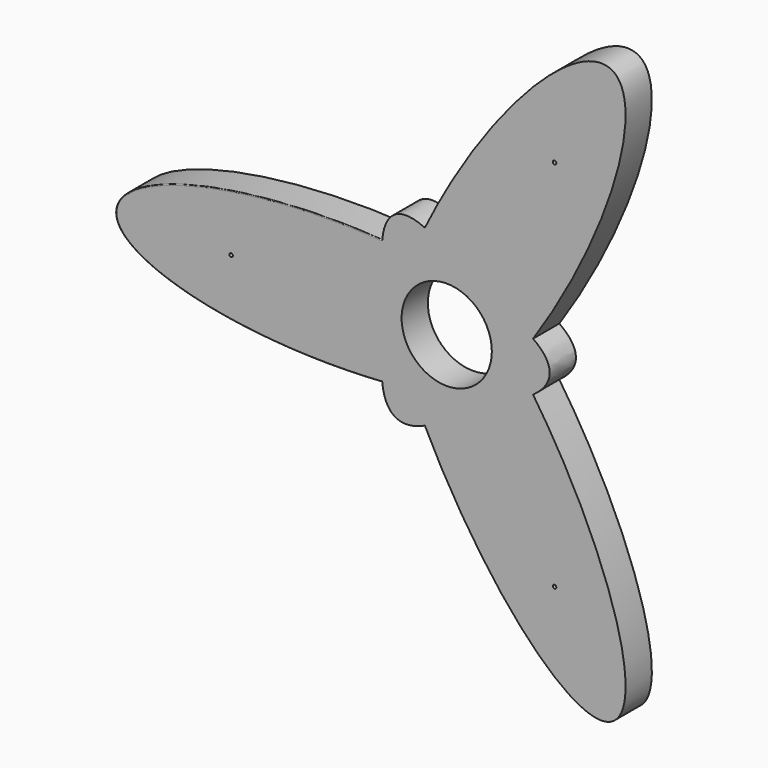
from build123d import *

# Parameters (mm, degrees)
F0_R     = 11
F0_R_2   = 279.4
F1_DEPTH = 203.2
F2_R     = 5.08


with BuildPart() as f1:
    # F0 (on Front) → F1 (new body)
    with BuildSketch(Plane.XZ):
        with BuildLine():
            add(Edge.make_bspline(
                [(1142.9615501258, -114.3779510258), (1245.7472762878, -41.1863168561), (1245.7472762878, 38.0692582474)],
                knots=[5.889466389, 5.889466389, 5.889466389, 6.2831853072, 6.2831853072, 6.2831853072], degree=2, weights=[1, 0.9806856728, 1]))
            add(Edge.make_bspline(
                [(1245.7472762878, 38.0692582474), (1245.7472762878, 117.3248333509), (1142.9615501258, 190.5164675206)],
                knots=[0, 0, 0, 0.3937189182, 0.3937189182, 0.3937189182], degree=2, weights=[1, 0.9806856728, 1]))
            add(Edge.make_bspline(
                [(1035.1117115223, 38.0692582474), (1089.7127136576, 111.4653325757), (1142.9615501258, 190.5164675206)],
                knots=[1.1955382149, 1.1955382149, 1.1955382149, 1.3406731889, 1.3406731889, 1.3406731889], degree=2, weights=[1, 0.9973681352, 1]))
            add(Edge.make_bspline(
                [(1142.9615501258, -114.3779510258), (1089.7127136576, -35.3268160809), (1035.1117115224, 38.0692582474)],
                knots=[4.9425121183, 4.9425121183, 4.9425121183, 5.0876470923, 5.0876470923, 5.0876470923], degree=2, weights=[1, 0.9973681352, 1]))
        make_face()
        with BuildLine():
            add(Edge.make_bspline(
                [(1035.1117115223, 38.0692582474), (1089.7127136576, 111.4653325757), (1142.9615501258, 190.5164675206)],
                knots=[1.1955382149, 1.1955382149, 1.1955382149, 1.3406731889, 1.3406731889, 1.3406731889], degree=2, weights=[1, 0.9973681352, 1]))
            add(Edge.make_bspline(
                [(1142.9615501258, 190.5164675206), (1021.3356442806, 277.1238121256), (781.6391771742, 338.5073699231)],
                knots=[0.3937189182, 0.3937189182, 0.3937189182, 0.8572367362, 0.8572367362, 0.8572367362], degree=2, weights=[1, 0.9732638973, 1]))
            add(Edge.make_bspline(
                [(1035.1117115224, 38.0692582474), (906.8375929399, 210.498634517), (781.6391771743, 338.5073699231)],
                knots=[5.0876470923, 5.0876470923, 5.0876470923, 5.4259485709, 5.4259485709, 5.4259485709], degree=2, weights=[1, 0.9857280914, 1]))
        make_face()
        with BuildLine():
            add(Edge.make_bspline(
                [(1142.9615501258, 190.5164675206), (1021.3356442806, 277.1238121256), (781.6391771742, 338.5073699231)],
                knots=[0.3937189182, 0.3937189182, 0.3937189182, 0.8572367362, 0.8572367362, 0.8572367362], degree=2, weights=[1, 0.9732638973, 1]))
            add(Edge.make_bspline(
                [(1142.9615501258, 190.5164675206), (2066.8933718666, 1562.149426371), (1632.8052788588, 1812.770303721), (1198.717185851, 2063.391181071), (472.814109689, 577.4262726536)],
                knots=[1.3406731889, 1.3406731889, 1.3406731889, 3.1415926536, 3.1415926536, 4.9425121183, 4.9425121183, 4.9425121183], degree=2, weights=[1, 0.6212497819, 1, 0.6212497819, 1]))
            add(Edge.make_bspline(
                [(781.6391771743, 338.5073699231), (608.6312231939, 515.3988207358), (472.814109689, 577.4262726536)],
                knots=[5.4259485709, 5.4259485709, 5.4259485709, 5.889466389, 5.889466389, 5.889466389], degree=2, weights=[1, 0.9732638973, 1]))
        make_face()
        with Locations((1275.7997997413, 1194.4186753089)):
            Circle(F0_R, mode=Mode.SUBTRACT)
        with BuildLine():
            add(Edge.make_bspline(
                [(472.814109689, -501.2877561588), (1198.717185851, -1987.2526645763), (1632.8052788588, -1736.6317872262), (2066.8933718666, -1486.0109098762), (1142.9615501258, -114.3779510258)],
                knots=[1.3406731889, 1.3406731889, 1.3406731889, 3.1415926536, 3.1415926536, 4.9425121183, 4.9425121183, 4.9425121183], degree=2, weights=[1, 0.6212497819, 1, 0.6212497819, 1]))
            add(Edge.make_bspline(
                [(781.6391771742, -262.3688534283), (1021.3356442806, -200.9852956308), (1142.9615501258, -114.3779510258)],
                knots=[5.4259485709, 5.4259485709, 5.4259485709, 5.889466389, 5.889466389, 5.889466389], degree=2, weights=[1, 0.9732638973, 1]))
            add(Edge.make_bspline(
                [(472.814109689, -501.2877561588), (608.6312231938, -439.260304241), (781.6391771743, -262.3688534283)],
                knots=[0.3937189182, 0.3937189182, 0.3937189182, 0.8572367362, 0.8572367362, 0.8572367362], degree=2, weights=[1, 0.9732638973, 1]))
        make_face()
        with Locations((1275.7997997413, -1118.2801588142)):
            Circle(F0_R, mode=Mode.SUBTRACT)
        with BuildLine():
            add(Edge.make_bspline(
                [(781.6391771742, -262.3688534283), (1021.3356442806, -200.9852956308), (1142.9615501258, -114.3779510258)],
                knots=[5.4259485709, 5.4259485709, 5.4259485709, 5.889466389, 5.889466389, 5.889466389], degree=2, weights=[1, 0.9732638973, 1]))
            add(Edge.make_bspline(
                [(1142.9615501258, -114.3779510258), (1089.7127136576, -35.3268160809), (1035.1117115224, 38.0692582474)],
                knots=[4.9425121183, 4.9425121183, 4.9425121183, 5.0876470923, 5.0876470923, 5.0876470923], degree=2, weights=[1, 0.9973681352, 1]))
            add(Edge.make_bspline(
                [(781.6391771743, -262.3688534283), (906.8375929399, -134.3601180223), (1035.1117115223, 38.0692582474)],
                knots=[0.8572367362, 0.8572367362, 0.8572367362, 1.1955382149, 1.1955382149, 1.1955382149], degree=2, weights=[1, 0.9857280914, 1]))
        make_face()
        with BuildLine():
            add(Edge.make_bspline(
                [(781.6391771742, 338.5073699231), (608.1811525235, 382.9280107866), (394.7158730241, 407.8019679923)],
                knots=[0.8572367362, 0.8572367362, 0.8572367362, 1.1955382149, 1.1955382149, 1.1955382149], degree=2, weights=[1, 0.9857280914, 1]))
            add(Edge.make_bspline(
                [(781.6391771743, 338.5073699231), (608.6312231939, 515.3988207358), (472.814109689, 577.4262726536)],
                knots=[5.4259485709, 5.4259485709, 5.4259485709, 5.889466389, 5.889466389, 5.889466389], degree=2, weights=[1, 0.9732638973, 1]))
            add(Edge.make_bspline(
                [(472.814109689, 577.4262726536), (430.9782368628, 491.7858600776), (394.7158730241, 407.8019679922)],
                knots=[4.9425121183, 4.9425121183, 4.9425121183, 5.0876470923, 5.0876470923, 5.0876470923], degree=2, weights=[1, 0.9973681352, 1]))
        make_face()
        with BuildLine():
            add(Edge.make_bspline(
                [(472.814109689, 577.4262726536), (430.9782368628, 491.7858600776), (394.7158730241, 407.8019679922)],
                knots=[4.9425121183, 4.9425121183, 4.9425121183, 5.0876470923, 5.0876470923, 5.0876470923], degree=2, weights=[1, 0.9973681352, 1]))
            add(Edge.make_bspline(
                [(472.814109689, 577.4262726536), (358.0354320725, 629.8455055714), (289.3980906413, 590.2177180197)],
                knots=[5.889466389, 5.889466389, 5.889466389, 6.2831853072, 6.2831853072, 6.2831853072], degree=2, weights=[1, 0.9806856728, 1]))
            add(Edge.make_bspline(
                [(289.3980906413, 590.2177180197), (220.7607492101, 550.5899304679), (208.7677977557, 424.9790633804)],
                knots=[0, 0, 0, 0.3937189182, 0.3937189182, 0.3937189182], degree=2, weights=[1, 0.9806856728, 1]))
            add(Edge.make_bspline(
                [(394.7158730241, 407.8019679923), (303.8525070501, 418.3897857493), (208.7677977557, 424.9790633804)],
                knots=[1.1955382149, 1.1955382149, 1.1955382149, 1.3406731889, 1.3406731889, 1.3406731889], degree=2, weights=[1, 0.9973681352, 1]))
        make_face()
        with BuildLine():
            add(Edge.make_bspline(
                [(472.814109689, -501.2877561588), (608.6312231938, -439.260304241), (781.6391771743, -262.3688534283)],
                knots=[0.3937189182, 0.3937189182, 0.3937189182, 0.8572367362, 0.8572367362, 0.8572367362], degree=2, weights=[1, 0.9732638973, 1]))
            add(Edge.make_bspline(
                [(394.7158730241, -331.6634514975), (608.1811525235, -306.7894942918), (781.6391771742, -262.3688534283)],
                knots=[5.0876470923, 5.0876470923, 5.0876470923, 5.4259485709, 5.4259485709, 5.4259485709], degree=2, weights=[1, 0.9857280914, 1]))
            add(Edge.make_bspline(
                [(394.7158730241, -331.6634514975), (430.9782368628, -415.6473435828), (472.814109689, -501.2877561588)],
                knots=[1.1955382149, 1.1955382149, 1.1955382149, 1.3406731889, 1.3406731889, 1.3406731889], degree=2, weights=[1, 0.9973681352, 1]))
        make_face()
        with BuildLine():
            add(Edge.make_bspline(
                [(289.3980906413, -514.0792015249), (358.0354320725, -553.7069890767), (472.814109689, -501.2877561588)],
                knots=[0, 0, 0, 0.3937189182, 0.3937189182, 0.3937189182], degree=2, weights=[1, 0.9806856728, 1]))
            add(Edge.make_bspline(
                [(394.7158730241, -331.6634514975), (430.9782368628, -415.6473435828), (472.814109689, -501.2877561588)],
                knots=[1.1955382149, 1.1955382149, 1.1955382149, 1.3406731889, 1.3406731889, 1.3406731889], degree=2, weights=[1, 0.9973681352, 1]))
            add(Edge.make_bspline(
                [(208.7677977557, -348.8405468856), (303.8525070501, -342.2512692545), (394.7158730241, -331.6634514975)],
                knots=[4.9425121183, 4.9425121183, 4.9425121183, 5.0876470923, 5.0876470923, 5.0876470923], degree=2, weights=[1, 0.9973681352, 1]))
            add(Edge.make_bspline(
                [(208.7677977557, -348.8405468856), (220.7607492101, -474.4514139731), (289.3980906413, -514.0792015249)],
                knots=[5.889466389, 5.889466389, 5.889466389, 6.2831853072, 6.2831853072, 6.2831853072], degree=2, weights=[1, 0.9806856728, 1]))
        make_face()
        with BuildLine():
            add(Edge.make_bspline(
                [(394.7158730241, 407.8019679922), (309.5247121071, 210.498634517), (261.2651032219, 38.0692582474)],
                knots=[5.0876470923, 5.0876470923, 5.0876470923, 5.4259485709, 5.4259485709, 5.4259485709], degree=2, weights=[1, 0.9857280914, 1]))
            add(Edge.make_bspline(
                [(394.7158730241, 407.8019679923), (303.8525070501, 418.3897857493), (208.7677977557, 424.9790633804)],
                knots=[1.1955382149, 1.1955382149, 1.1955382149, 1.3406731889, 1.3406731889, 1.3406731889], degree=2, weights=[1, 0.9973681352, 1]))
            add(Edge.make_bspline(
                [(208.7677977557, 424.9790633804), (194.5765900961, 276.3442668575), (261.2651032219, 38.0692582474)],
                knots=[0.3937189182, 0.3937189182, 0.3937189182, 0.8572367362, 0.8572367362, 0.8572367362], degree=2, weights=[1, 0.9732638973, 1]))
        make_face()
        with BuildLine():
            add(Edge.make_bspline(
                [(208.7677977557, -348.8405468856), (303.8525070501, -342.2512692545), (394.7158730241, -331.6634514975)],
                knots=[4.9425121183, 4.9425121183, 4.9425121183, 5.0876470923, 5.0876470923, 5.0876470923], degree=2, weights=[1, 0.9973681352, 1]))
            add(Edge.make_bspline(
                [(261.2651032219, 38.0692582474), (309.5247121071, -134.3601180222), (394.7158730241, -331.6634514975)],
                knots=[0.8572367362, 0.8572367362, 0.8572367362, 1.1955382149, 1.1955382149, 1.1955382149], degree=2, weights=[1, 0.9857280914, 1]))
            add(Edge.make_bspline(
                [(261.2651032219, 38.0692582474), (194.5765900961, -200.2057503628), (208.7677977557, -348.8405468856)],
                knots=[5.4259485709, 5.4259485709, 5.4259485709, 5.889466389, 5.889466389, 5.889466389], degree=2, weights=[1, 0.9732638973, 1]))
        make_face()
        with BuildLine():
            add(Edge.make_bspline(
                [(208.7677977557, 424.9790633804), (194.5765900961, 276.3442668575), (261.2651032219, 38.0692582474)],
                knots=[0.3937189182, 0.3937189182, 0.3937189182, 0.8572367362, 0.8572367362, 0.8572367362], degree=2, weights=[1, 0.9732638973, 1]))
            add(Edge.make_bspline(
                [(208.7677977557, 424.9790633804), (-1441.0671001471, 539.3110129475), (-1441.0671001471, 38.0692582474), (-1441.0671001471, -463.1724964527), (208.7677977557, -348.8405468856)],
                knots=[1.3406731889, 1.3406731889, 1.3406731889, 3.1415926536, 3.1415926536, 4.9425121183, 4.9425121183, 4.9425121183], degree=2, weights=[1, 0.6212497819, 1, 0.6212497819, 1]))
            add(Edge.make_bspline(
                [(261.2651032219, 38.0692582474), (194.5765900961, -200.2057503628), (208.7677977557, -348.8405468856)],
                knots=[5.4259485709, 5.4259485709, 5.4259485709, 5.889466389, 5.889466389, 5.889466389], degree=2, weights=[1, 0.9732638973, 1]))
        make_face()
        with Locations((-727.056141912, 38.0692582474)):
            Circle(F0_R, mode=Mode.SUBTRACT)
        with BuildLine():
            add(Edge.make_bspline(
                [(1035.1117115224, 38.0692582474), (906.8375929399, 210.498634517), (781.6391771743, 338.5073699231)],
                knots=[5.0876470923, 5.0876470923, 5.0876470923, 5.4259485709, 5.4259485709, 5.4259485709], degree=2, weights=[1, 0.9857280914, 1]))
            add(Edge.make_bspline(
                [(781.6391771742, 338.5073699231), (608.1811525235, 382.9280107866), (394.7158730241, 407.8019679923)],
                knots=[0.8572367362, 0.8572367362, 0.8572367362, 1.1955382149, 1.1955382149, 1.1955382149], degree=2, weights=[1, 0.9857280914, 1]))
            add(Edge.make_bspline(
                [(394.7158730241, 407.8019679922), (309.5247121071, 210.498634517), (261.2651032219, 38.0692582474)],
                knots=[5.0876470923, 5.0876470923, 5.0876470923, 5.4259485709, 5.4259485709, 5.4259485709], degree=2, weights=[1, 0.9857280914, 1]))
            add(Edge.make_bspline(
                [(261.2651032219, 38.0692582474), (309.5247121071, -134.3601180222), (394.7158730241, -331.6634514975)],
                knots=[0.8572367362, 0.8572367362, 0.8572367362, 1.1955382149, 1.1955382149, 1.1955382149], degree=2, weights=[1, 0.9857280914, 1]))
            add(Edge.make_bspline(
                [(394.7158730241, -331.6634514975), (608.1811525235, -306.7894942918), (781.6391771742, -262.3688534283)],
                knots=[5.0876470923, 5.0876470923, 5.0876470923, 5.4259485709, 5.4259485709, 5.4259485709], degree=2, weights=[1, 0.9857280914, 1]))
            add(Edge.make_bspline(
                [(781.6391771743, -262.3688534283), (906.8375929399, -134.3601180223), (1035.1117115223, 38.0692582474)],
                knots=[0.8572367362, 0.8572367362, 0.8572367362, 1.1955382149, 1.1955382149, 1.1955382149], degree=2, weights=[1, 0.9857280914, 1]))
        make_face()
        with Locations((608.1811525235, 38.0692582474)):
            Circle(F0_R_2, mode=Mode.SUBTRACT)
    extrude(amount=F1_DEPTH)

    # F2
    f2_edges = [f1.edges().sort_by_distance(p)[0] for p in [
        (-1441.0671, -203.2, 38.069258),
    ]]
    fillet(f2_edges, radius=F2_R)


solid = f1.part
